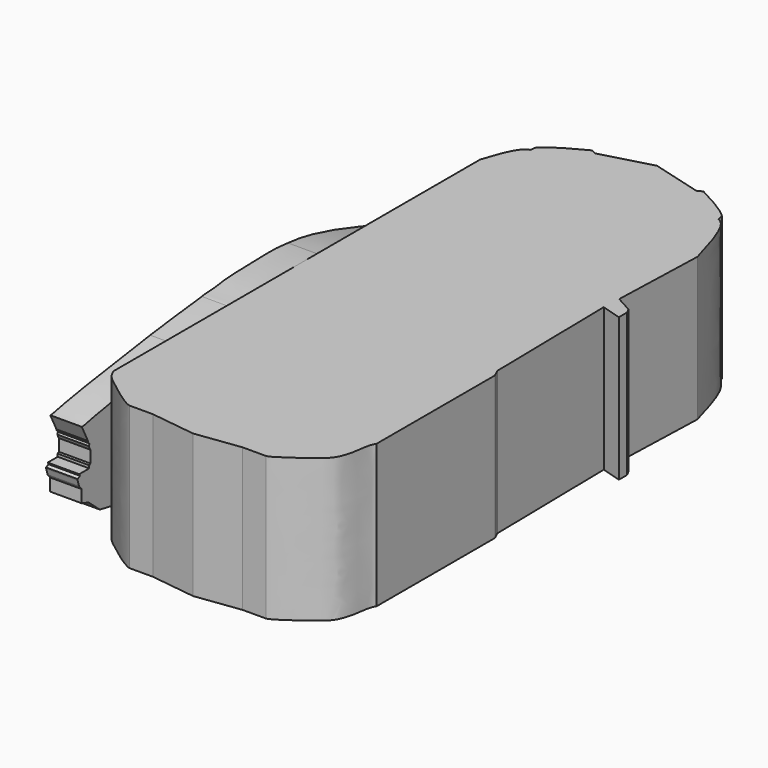
from build123d import *

# Parameters (mm, degrees)
F0_W     = 464.551
F0_H     = 113.6
F1_DEPTH = 113.25
F2_DEPTH = 113.25
F4_DEPTH = 25
F6_DEPTH = 1000


with BuildPart() as f1:
    # F0 (on Right) → F1 (new body)
    with BuildSketch(Plane.YZ):
        with Locations((0, 56.8)):
            Rectangle(F0_W, F0_H)
    extrude(amount=F1_DEPTH)

    # F2 (add): a face of the model
    f2_faces = [f1.faces().sort_by_distance(p)[0] for p in [
        (0, 0, 56.8),
    ]]
    extrude(f2_faces, amount=F2_DEPTH)

    # F3 (on face) → F4 (cut)
    with BuildSketch(Plane(origin=(-113.25, 0, 0), x_dir=(0, -1, 0), z_dir=(-1, 0, 0))):
        with BuildLine():
            Line((-232.2755, 113.6), (-232.2755, 32.8185763762))
            add(Edge.make_bspline(
                [(-232.2755, 32.8185763762), (-231.8790980509, 34.173098972), (-231.4615017526, 35.2897108989), (-231.1046542652, 36.061558603)],
                knots=[0.3164856699, 0.3164856699, 0.3164856699, 0.3164856699, 0.340416374, 0.340416374, 0.340416374, 0.340416374], degree=3))
            add(Edge.make_bspline(
                [(-231.1046542652, 36.061558603), (-231.1037416795, 36.0635324916), (-231.1028294911, 36.0655041254), (-231.1019176999, 36.0674735084)],
                knots=[0.340416374, 0.340416374, 0.340416374, 0.340416374, 0.3404775733, 0.3404775733, 0.3404775733, 0.3404775733], degree=3))
            add(Edge.make_bspline(
                [(-231.1019176999, 36.0674735084), (-230.6559874539, 37.3781955492), (-230.2235967105, 37.6932665807), (-229.7431129588, 38.2673442747), (-229.7240369276, 38.2904159632)],
                knots=[0.3710065635, 0.3710065635, 0.3710065635, 0.3710065635, 0.408928644, 0.410487131, 0.410487131, 0.410487131, 0.410487131], degree=3))
            add(Edge.make_bspline(
                [(-229.7240369276, 38.2904159632), (-229.3831871996, 38.9468266155), (-228.9939173404, 40.7418408458), (-222.7621322692, 45.1945330228), (-218.9446701646, 47.5596041628)],
                knots=[0.3837612534, 0.3837612534, 0.3837612534, 0.3837612534, 0.4345564552, 0.4775666683, 0.4775666683, 0.4775666683, 0.4775666683], degree=3))
            add(Edge.make_bspline(
                [(-218.9446701646, 47.5596041628), (-201.1108713778, 59.1756051595), (-159.2165627136, 79.5233669449), (-124.8394856244, 78.5623382324)],
                knots=[0.5003760226, 0.5003760226, 0.5003760226, 0.5003760226, 0.7066174583, 0.7066174583, 0.7066174583, 0.7066174583], degree=3))
            Line((-124.8394856244, 78.5623382324), (-124.8128838181, 78.5711071926))
            add(Edge.make_bspline(
                [(-124.8128838181, 78.5711071926), (-95.4129047028, 89.3393301028), (-52.7253294089, 104.695750439), (-18.6634613097, 111.2791553675), (-8.6977606118, 111.9964196387)],
                knots=[0, 0, 0, 0, 0.4399174375, 0.6645176817, 0.6645176817, 0.6645176817, 0.6645176817], degree=3))
            add(Edge.make_bspline(
                [(-8.6977606118, 111.9964196387), (2.6332697065, 113.6), (20.4424923427, 112.7872208771), (35.963276732, 112.6549982749), (45.5451939753, 112.3018279721), (56.6888041617, 111.6409761871), (64.2975464247, 109.951929701), (75.0365459893, 109.9324073647), (76.5711785486, 109.2785894871)],
                knots=[0, 0, 0, 0, 0.2490636409, 0.4235691057, 0.5634534133, 0.7107894117, 0.8474028434, 1, 1, 1, 1], degree=3))
            add(Edge.make_bspline(
                [(76.5711785486, 109.2785894871), (98.8196080664, 107.0355331865), (101.2230982613, 106.3033664287), (121.0916796929, 104.1045469497), (127.9400074251, 103.1173849293)],
                knots=[0, 0, 0, 0, 0.350874071, 0.5612199162, 0.5612199162, 0.5612199162, 0.5612199162], degree=3))
            add(Edge.make_bspline(
                [(127.9400074251, 103.1173849293), (153.8156108236, 99.4933517824), (189.8635745439, 94.1924701653), (199.3642186335, 92.2866301463), (217.3858562933, 89.420523582), (224.3752265839, 87.4593358123), (226.7716812547, 87.4656452566), (227.0337724394, 87.4753445387)],
                knots=[0, 0, 0, 0, 0.3930552732, 0.5481620816, 0.755041436, 0.9024722065, 0.9211456239, 0.9211456239, 0.9211456239, 0.9211456239], degree=3))
            Line((227.0337724394, 87.4753445387), (220.8725305078, 75.1084685326))
            Line((220.8725305078, 75.1084685326), (220.8725305078, 74.2925181985))
            Line((220.8725305078, 74.2925181985), (219.4038273609, 72.7422088385))
            Line((219.4038273609, 72.7422088385), (220.1381863869, 71.1918994784))
            Line((220.1381863869, 71.1918994784), (218.5948135174, 68.0700615048))
            Line((218.5948135174, 68.0700615048), (218.5948135174, 58.5093386471))
            Line((218.5948135174, 58.5093386471), (219.6228446281, 57.5841069222))
            Line((219.6228446281, 57.5841069222), (219.6228446281, 55.4252304137))
            Line((219.6228446281, 55.4252304137), (225.688257984, 55.4252304137))
            Line((225.688257984, 55.4252304137), (229.594791106, 55.4252304137))
            Line((229.594791106, 55.4252304137), (228.8092614925, 53.9363473654))
            Line((228.8092614925, 53.9363473654), (231.2004830437, 52.6747470382))
            Line((231.2004830437, 52.6747470382), (231.2004830437, 51.8779531121))
            Line((231.2004830437, 51.8779531121), (229.7012301004, 47.0750369132))
            Line((229.7012301004, 47.0750369132), (227.1657975233, 44.0031215549))
            Line((227.1657975233, 44.0031215549), (227.1657975233, 34.1228358448))
            Line((227.1657975233, 34.1228358448), (220.304498247, 31.9272167981))
            Line((220.304498247, 31.9272167981), (209.0519459761, 22.3213806748))
            Line((209.0519459761, 22.3213806748), (184.955375434, 17.8825389594))
            Line((184.955375434, 17.8825389594), (181.8208045852, 17.8825389594))
            add(Edge.make_bspline(
                [(109.7462345314, 11.3512530682), (105.13303124, 21.9971068237), (102.3295920912, 31.0067949184), (104.3007691763, 39.3500479436), (106.5787886857, 48.4665274974), (109.1198933454, 54.6206926313), (110.6540323122, 58.1162692133), (114.1247970317, 64.2584038543), (121.206458876, 69.1007924931), (128.0023361028, 72.5621948893), (135.7815625135, 75.1533703094), (158.4659606039, 76.2432867824), (173.9848172528, 69.3513817398), (182.8990728751, 48.3394334811), (186.6540110233, 40.7480202803), (182.5457507186, 21.0076564597), (181.8208045852, 17.8825389594)],
                knots=[0, 0, 0, 0, 0.0987938644, 0.1562912272, 0.2214221262, 0.2754761052, 0.3164249447, 0.3714453076, 0.4337725763, 0.4910116539, 0.5514503521, 0.6509165337, 0.7371979116, 0.8298327622, 0.929885825, 0.9556923225, 0.9556923225, 0.9556923225, 0.9556923225], degree=3))
            Line((109.7462345314, 11.3512530682), (-44.88848494, 8.9413357289))
            add(Edge.make_bspline(
                [(-44.88848494, 8.9413357289), (-43.1857559899, 5.9007342453), (-41.5231174, 2.9081292823), (-39.890128567, 0)],
                knots=[0.9375411424, 0.9375411424, 0.9375411424, 0.9375411424, 0.959328761, 0.959328761, 0.959328761, 0.959328761], degree=3))
            Line((-39.890128567, 0), (182.4303716421, 0))
            Line((182.4303716421, 0), (232.2755, 0))
            Line((232.2755, 0), (232.2755, 113.6))
            Line((232.2755, 113.6), (-232.2755, 113.6))
        make_face()
        with BuildLine():
            add(Edge.make_bspline(
                [(-164.6185908859, 5.2917431583), (-165.0713665181, 6.1458001934), (-165.5417803562, 7.0626109679), (-165.9595008133, 7.8887262308)],
                knots=[0.0253739484, 0.0253739484, 0.0253739484, 0.0253739484, 0.0325818946, 0.0325818946, 0.0325818946, 0.0325818946], degree=3))
            add(Edge.make_bspline(
                [(-164.6185908829, 5.2917431614), (-176.0597302488, 5.0024554897), (-221.4994853953, -2.2050957763), (-231.4882447651, 12.8488706649), (-232.2755, 14.7370494299)],
                knots=[0.0067884722, 0.0067884722, 0.0067884722, 0.0067884722, 0.2079627726, 0.2341336285, 0.2341336285, 0.2341336285, 0.2341336285], degree=3))
            Line((-232.2755, 14.7370494299), (-232.2755, 0))
            Line((-232.2755, 0), (-199.7243613005, 0))
            Line((-199.7243613005, 0), (-108.776524663, 0))
            add(Edge.make_bspline(
                [(-99.5009951625, 8.0902226298), (-100.0590209927, 7.5668730715), (-101.5069269475, 6.5632143557), (-103.3306144836, 6.7731347239), (-108.7701587892, 1.0011318839), (-108.776524663, 0)],
                knots=[0.9080949913, 0.9080949913, 0.9080949913, 0.9080949913, 0.9266826271, 0.9527213106, 1, 1, 1, 1], degree=3))
            add(Edge.make_bspline(
                [(-165.999836251, 7.9685384826), (-166.1315589651, 8.2293162171), (-168.3484257522, 12.6415430944), (-167.9805882713, 12.4600804675), (-169.7120256252, 17.9777869169), (-169.9426153794, 22.5907371267), (-169.5424098093, 28.9978956361), (-168.7921487837, 37.5297393179), (-166.0332983923, 49.9674844075), (-151.3616999612, 63.434506998), (-134.8432776987, 68.1280958415), (-117.8900740705, 65.973738886), (-105.2585534529, 57.8915639024), (-99.8095863375, 46.4784476464), (-97.2456192191, 38.6154807096), (-96.7354298507, 35.5495889525), (-95.4008258624, 29.1857470823), (-94.3373664851, 24.3061446971), (-95.2367782113, 18.2710500862), (-97.0664400304, 13.2465953537), (-97.7713663779, 9.980297143), (-99.1001790926, 8.4661315964), (-99.5009951625, 8.0902226298)],
                knots=[0.0328148598, 0.0328148598, 0.0328148598, 0.0328148598, 0.0351068846, 0.0730884918, 0.1078890541, 0.1446769101, 0.1863042014, 0.2349017732, 0.2935240518, 0.3663928625, 0.4352730595, 0.5031486338, 0.5664856863, 0.6257751938, 0.6724005796, 0.7019430205, 0.7436099057, 0.781676286, 0.8223597691, 0.8611079585, 0.894743955, 0.9080949913, 0.9080949913, 0.9080949913, 0.9080949913], degree=3))
            add(Edge.make_bspline(
                [(-165.9595008133, 7.8887262308), (-165.9730017954, 7.9154267842), (-165.9864477329, 7.9420325951), (-165.999836251, 7.9685384826)],
                knots=[0.0325818946, 0.0325818946, 0.0325818946, 0.0325818946, 0.0328148598, 0.0328148598, 0.0328148598, 0.0328148598], degree=3))
        make_face()
        with BuildLine():
            add(Edge.make_bspline(
                [(-163.5608168843, 5.2993261556), (-163.8792031032, 5.3043338554), (-164.2325184235, 5.3015049516), (-164.6185908829, 5.2917431614)],
                knots=[0, 0, 0, 0, 0.0067884722, 0.0067884722, 0.0067884722, 0.0067884722], degree=3))
            add(Edge.make_bspline(
                [(-163.5608168843, 5.2993261556), (-161.649380445, 0.0563780767), (-163.0246964147, 2.285228034), (-164.6185908859, 5.2917431583)],
                knots=[0, 0, 0, 0, 0.0253739484, 0.0253739484, 0.0253739484, 0.0253739484], degree=3))
        make_face(mode=Mode.SUBTRACT)
        with BuildLine():
            Line((-47.060206555, 8.9074903571), (-99.5009951625, 8.0902226298))
            add(Edge.make_bspline(
                [(-99.5009951625, 8.0902226298), (-100.0590209927, 7.5668730715), (-101.5069269475, 6.5632143557), (-103.3306144836, 6.7731347239), (-108.7701587892, 1.0011318839), (-108.776524663, 0)],
                knots=[0.9080949913, 0.9080949913, 0.9080949913, 0.9080949913, 0.9266826271, 0.9527213106, 1, 1, 1, 1], degree=3))
            Line((-108.776524663, 0), (-42.181071883, 0))
            add(Edge.make_bspline(
                [(-47.060206555, 8.9074903571), (-45.4160903787, 5.8952523745), (-43.7940471019, 2.9154941638), (-42.181071883, 0)],
                knots=[0.9352203433, 0.9352203433, 0.9352203433, 0.9352203433, 0.9579142214, 0.9579142214, 0.9579142214, 0.9579142214], degree=3))
        make_face()
        with BuildLine():
            add(Edge.make_bspline(
                [(-164.6185908829, 5.2917431614), (-176.0597302488, 5.0024554897), (-221.4994853953, -2.2050957763), (-231.4882447651, 12.8488706649), (-232.2755, 14.7370494299)],
                knots=[0.0067884722, 0.0067884722, 0.0067884722, 0.0067884722, 0.2079627726, 0.2341336285, 0.2341336285, 0.2341336285, 0.2341336285], degree=3))
            add(Edge.make_bspline(
                [(-164.6185908859, 5.2917431583), (-165.0713665181, 6.1458001934), (-165.5417803562, 7.0626109679), (-165.9595008133, 7.8887262308)],
                knots=[0.0253739484, 0.0253739484, 0.0253739484, 0.0253739484, 0.0325818946, 0.0325818946, 0.0325818946, 0.0325818946], degree=3))
            Line((-165.9595008133, 7.8887262308), (-173.761184881, 7.8887262308))
            add(Edge.make_bspline(
                [(-173.761184881, 7.8887262308), (-184.52015401, 6.7813550005), (-212.0861099631, 1.0960000393), (-224.4535929193, 8.6120162565)],
                knots=[0.0748722313, 0.0748722313, 0.0748722313, 0.0748722313, 0.2385609184, 0.2385609184, 0.2385609184, 0.2385609184], degree=3))
            add(Edge.make_bspline(
                [(-224.4535929198, 8.6120162548), (-225.593511103, 8.6582821597), (-226.9193272524, 8.9787715082), (-228.5662179841, 10.1463577013), (-228.0852725306, 10.5369179466), (-227.5320876257, 11.1132782623)],
                knots=[0.0190189348, 0.0190189348, 0.0190189348, 0.0190189348, 0.1288080398, 0.2164411512, 0.2955399174, 0.2955399174, 0.2955399174, 0.2955399174], degree=3))
            add(Edge.make_bspline(
                [(-227.5320876257, 11.1132782623), (-229.4142893106, 13.1628592742), (-230.626158224, 15.7357057729), (-231.3651247853, 18.4617653178)],
                knots=[0.2540536411, 0.2540536411, 0.2540536411, 0.2540536411, 0.287279567, 0.287279567, 0.287279567, 0.287279567], degree=3))
            add(Edge.make_bspline(
                [(-231.3651247856, 18.4617653194), (-231.6664931574, 18.3945211663), (-231.970246093, 18.3269098965), (-232.2755, 18.2591101898)],
                knots=[0.904683008, 0.904683008, 0.904683008, 0.904683008, 0.9170355344, 0.9170355344, 0.9170355344, 0.9170355344], degree=3))
            Line((-232.2755, 18.2591101898), (-232.2755, 14.7370494299))
        make_face()
        with BuildLine():
            add(Edge.make_bspline(
                [(-231.3651247853, 18.4617653178), (-231.8634715688, 20.3001746276), (-232.1467456858, 22.2082641541), (-232.2755, 24.0725370259)],
                knots=[0.287279567, 0.287279567, 0.287279567, 0.287279567, 0.30968658, 0.30968658, 0.30968658, 0.30968658], degree=3))
            add(Edge.make_bspline(
                [(-219.9768019121, 22.3368026759), (-220.4194158688, 22.4551950684), (-222.5269750091, 20.7593592711), (-222.0798182071, 20.5782839942), (-226.6219868008, 19.5200989952), (-231.3651247856, 18.4617653194)],
                knots=[0.5724422355, 0.5724422355, 0.5724422355, 0.5724422355, 0.6920254287, 0.7102706449, 0.904683008, 0.904683008, 0.904683008, 0.904683008], degree=3))
            add(Edge.make_bspline(
                [(-231.1042252985, 36.0606825889), (-230.5188300394, 34.8653239168), (-228.1407765352, 30.8516739145), (-225.1993287881, 26.8897443239), (-222.8176913923, 24.1323083158), (-220.2737508162, 22.4397358959), (-219.9768019121, 22.3368026759)],
                knots=[5.26887e-05, 5.26887e-05, 5.26887e-05, 5.26887e-05, 0.2157019808, 0.4186074107, 0.6166635747, 0.7051916224, 0.7051916224, 0.7051916224, 0.7051916224], degree=3))
            add(Edge.make_bspline(
                [(-232.2755, 29.1774376338), (-232.079015574, 32.1619360955), (-231.574978086, 34.6715181224), (-231.1052089772, 36.0577842723), (-231.1042252985, 36.0606825889)],
                knots=[0.3310073569, 0.3310073569, 0.3310073569, 0.3310073569, 0.3708575256, 0.3709411582, 0.3709411582, 0.3709411582, 0.3709411582], degree=3))
            Line((-232.2755, 29.1774376338), (-232.2755, 24.0725370259))
        make_face()
        with BuildLine():
            add(Edge.make_bspline(
                [(-173.761184881, 7.8887262308), (-184.52015401, 6.7813550005), (-212.0861099631, 1.0960000393), (-224.4535929193, 8.6120162565)],
                knots=[0.0748722313, 0.0748722313, 0.0748722313, 0.0748722313, 0.2385609184, 0.2385609184, 0.2385609184, 0.2385609184], degree=3))
            Line((-173.761184881, 7.8887262308), (-214.1551375389, 7.8887262308))
            Line((-214.1551375389, 7.8887262308), (-223.8230854273, 8.5997134447))
            add(Edge.make_bspline(
                [(-223.8230854273, 8.5997134447), (-224.0465712552, 8.5999469107), (-224.2561231466, 8.6040015412), (-224.4535929198, 8.6120162548)],
                knots=[0, 0, 0, 0, 0.0190189348, 0.0190189348, 0.0190189348, 0.0190189348], degree=3))
        make_face()
        with BuildLine():
            add(Edge.make_bspline(
                [(-218.9446701646, 47.5596041628), (-200.5086110348, 58.9814834606), (-159.678620058, 77.9481915129), (-126.6516175068, 77.9649911165)],
                knots=[0.4775666683, 0.4775666683, 0.4775666683, 0.4775666683, 0.6852802774, 0.6852802774, 0.6852802774, 0.6852802774], degree=3))
            Line((-126.6516175068, 77.9649911165), (-124.8394856244, 78.5623382324))
            add(Edge.make_bspline(
                [(-218.9446701646, 47.5596041628), (-201.1108713778, 59.1756051595), (-159.2165627136, 79.5233669449), (-124.8394856244, 78.5623382324)],
                knots=[0.5003760226, 0.5003760226, 0.5003760226, 0.5003760226, 0.7066174583, 0.7066174583, 0.7066174583, 0.7066174583], degree=3))
        make_face()
        with BuildLine():
            add(Edge.make_bspline(
                [(-219.9768019121, 22.3368026759), (-220.4194158688, 22.4551950684), (-222.5269750091, 20.7593592711), (-222.0798182071, 20.5782839942), (-226.6219868008, 19.5200989952), (-231.3651247856, 18.4617653194)],
                knots=[0.5724422355, 0.5724422355, 0.5724422355, 0.5724422355, 0.6920254287, 0.7102706449, 0.904683008, 0.904683008, 0.904683008, 0.904683008], degree=3))
            add(Edge.make_bspline(
                [(-227.5320876257, 11.1132782623), (-229.4142893106, 13.1628592742), (-230.626158224, 15.7357057729), (-231.3651247853, 18.4617653178)],
                knots=[0.2540536411, 0.2540536411, 0.2540536411, 0.2540536411, 0.287279567, 0.287279567, 0.287279567, 0.287279567], degree=3))
            add(Edge.make_bspline(
                [(-227.5320876257, 11.1132782623), (-227.400035455, 11.250862694), (-225.2045570672, 13.5818888158), (-219.0909408032, 21.9856806014), (-219.9598966124, 22.3312334306)],
                knots=[0.2955399174, 0.2955399174, 0.2955399174, 0.2955399174, 0.3144217844, 0.5708529783, 0.5708529783, 0.5708529783, 0.5708529783], degree=3))
            add(Edge.make_bspline(
                [(-219.9768019121, 22.3368026759), (-219.9709772016, 22.3347836208), (-219.9653405958, 22.3329261306), (-219.9598966124, 22.3312334306)],
                knots=[0.7051916224, 0.7051916224, 0.7051916224, 0.7051916224, 0.7069281172, 0.7069281172, 0.7069281172, 0.7069281172], degree=3))
        make_face()
        with BuildLine():
            Line((-44.88848494, 8.9413357289), (-47.060206555, 8.9074903571))
            add(Edge.make_bspline(
                [(-47.060206555, 8.9074903571), (-45.4160903787, 5.8952523745), (-43.7940471019, 2.9154941638), (-42.181071883, 0)],
                knots=[0.9352203433, 0.9352203433, 0.9352203433, 0.9352203433, 0.9579142214, 0.9579142214, 0.9579142214, 0.9579142214], degree=3))
            Line((-42.181071883, 0), (-39.890128567, 0))
            add(Edge.make_bspline(
                [(-44.88848494, 8.9413357289), (-43.1857559899, 5.9007342453), (-41.5231174, 2.9081292823), (-39.890128567, 0)],
                knots=[0.9375411424, 0.9375411424, 0.9375411424, 0.9375411424, 0.959328761, 0.959328761, 0.959328761, 0.959328761], degree=3))
        make_face()
        with BuildLine():
            add(Edge.make_bspline(
                [(-229.7240369276, 38.2904159632), (-229.3831871996, 38.9468266155), (-228.9939173404, 40.7418408458), (-222.7621322692, 45.1945330228), (-218.9446701646, 47.5596041628)],
                knots=[0.3837612534, 0.3837612534, 0.3837612534, 0.3837612534, 0.4345564552, 0.4775666683, 0.4775666683, 0.4775666683, 0.4775666683], degree=3))
            add(Edge.make_bspline(
                [(-229.7240369276, 38.2904159632), (-228.9042852099, 39.2818725235), (-227.5337806085, 41.62901739), (-220.9262489428, 46.2689076972), (-218.9446701646, 47.5596041628)],
                knots=[0.410487131, 0.410487131, 0.410487131, 0.410487131, 0.4774597805, 0.5003760226, 0.5003760226, 0.5003760226, 0.5003760226], degree=3))
        make_face()
        with BuildLine():
            add(Edge.make_bspline(
                [(-163.5608168843, 5.2993261556), (-161.649380445, 0.0563780767), (-163.0246964147, 2.285228034), (-164.6185908859, 5.2917431583)],
                knots=[0, 0, 0, 0, 0.0253739484, 0.0253739484, 0.0253739484, 0.0253739484], degree=3))
            add(Edge.make_bspline(
                [(-163.5608168843, 5.2993261556), (-163.8792031032, 5.3043338554), (-164.2325184235, 5.3015049516), (-164.6185908829, 5.2917431614)],
                knots=[0, 0, 0, 0, 0.0067884722, 0.0067884722, 0.0067884722, 0.0067884722], degree=3))
        make_face()
        with BuildLine():
            Line((-232.2755, 24.0725370259), (-232.2755, 18.2591101898))
            add(Edge.make_bspline(
                [(-231.3651247856, 18.4617653194), (-231.6664931574, 18.3945211663), (-231.970246093, 18.3269098965), (-232.2755, 18.2591101898)],
                knots=[0.904683008, 0.904683008, 0.904683008, 0.904683008, 0.9170355344, 0.9170355344, 0.9170355344, 0.9170355344], degree=3))
            add(Edge.make_bspline(
                [(-231.3651247853, 18.4617653178), (-231.8634715688, 20.3001746276), (-232.1467456858, 22.2082641541), (-232.2755, 24.0725370259)],
                knots=[0.287279567, 0.287279567, 0.287279567, 0.287279567, 0.30968658, 0.30968658, 0.30968658, 0.30968658], degree=3))
        make_face()
        with BuildLine():
            add(Edge.make_bspline(
                [(-232.2755, 32.8185763762), (-231.8790980509, 34.173098972), (-231.4615017526, 35.2897108989), (-231.1046542652, 36.061558603)],
                knots=[0.3164856699, 0.3164856699, 0.3164856699, 0.3164856699, 0.340416374, 0.340416374, 0.340416374, 0.340416374], degree=3))
            Line((-232.2755, 32.8185763762), (-232.2755, 29.1774376338))
            add(Edge.make_bspline(
                [(-232.2755, 29.1774376338), (-232.079015574, 32.1619360955), (-231.574978086, 34.6715181224), (-231.1052089772, 36.0577842723), (-231.1042252985, 36.0606825889)],
                knots=[0.3310073569, 0.3310073569, 0.3310073569, 0.3310073569, 0.3708575256, 0.3709411582, 0.3709411582, 0.3709411582, 0.3709411582], degree=3))
            add(Edge.make_bspline(
                [(-231.1046542652, 36.061558603), (-231.1045113145, 36.0612666504), (-231.1043683256, 36.0609746457), (-231.1042252985, 36.0606825889)],
                knots=[0, 0, 0, 0, 5.26887e-05, 5.26887e-05, 5.26887e-05, 5.26887e-05], degree=3))
        make_face()
        with BuildLine():
            add(Edge.make_bspline(
                [(-231.1046542652, 36.061558603), (-231.1037416795, 36.0635324916), (-231.1028294911, 36.0655041254), (-231.1019176999, 36.0674735084)],
                knots=[0.340416374, 0.340416374, 0.340416374, 0.340416374, 0.3404775733, 0.3404775733, 0.3404775733, 0.3404775733], degree=3))
            add(Edge.make_bspline(
                [(-231.1046542652, 36.061558603), (-231.1045113145, 36.0612666504), (-231.1043683256, 36.0609746457), (-231.1042252985, 36.0606825889)],
                knots=[0, 0, 0, 0, 5.26887e-05, 5.26887e-05, 5.26887e-05, 5.26887e-05], degree=3))
            add(Edge.make_bspline(
                [(-231.1042252985, 36.0606825889), (-231.1034560076, 36.0629492317), (-231.1026868082, 36.0652128694), (-231.1019176999, 36.0674735084)],
                knots=[0.3709411582, 0.3709411582, 0.3709411582, 0.3709411582, 0.3710065635, 0.3710065635, 0.3710065635, 0.3710065635], degree=3))
        make_face()
    extrude(amount=-F4_DEPTH, mode=Mode.SUBTRACT)

    # F5 (on face) → F6 (cut)
    with BuildSketch(Plane.XY.offset(113.6)):
        with BuildLine():
            add(Edge.make_bspline(
                [(98.4679684043, 150.3394693136), (92.97439072, 169.757588614), (87.4808130356, 189.1757079143), (80.6744733231, 195.6006419142)],
                knots=[0, 0, 0, 0, 0.3368607946, 0.3368607946, 0.3368607946, 0.3368607946], degree=3))
            Line((98.4679684043, 150.3394693136), (96.0445478559, 75.8095905185))
            Line((96.0445478559, 75.8095905185), (109.0543940663, 68.6613246799))
            Line((109.0543940663, 68.6613246799), (111.0559105873, 64.801260829))
            Line((111.0559105873, 64.801260829), (111.0559105873, 56.6522367299))
            Line((111.0559105873, 56.6522367299), (95.3297168016, 61.3700933754))
            Line((95.3297168016, 61.3700933754), (97.2140729427, -46.5304255486))
            Line((97.2140729427, -46.5304255486), (99.9343246222, -52.4809621274))
            Line((99.9343246222, -52.4809621274), (99.9343246222, -76.1131048203))
            Line((99.9343246222, -76.1131048203), (99.9343246222, -169.918820262))
            add(Edge.make_bspline(
                [(99.9343246222, -169.918820262), (97.4321093028, -173.1361196506), (96.4461367368, -184.839463119), (94.8029562123, -191.1416171803), (91.5085392438, -202.0027756883), (79.6216278842, -210.368717206), (70.4898681676, -217.4342853568), (68.7864026452, -218.5316457264), (60.0496902937, -224.5997639162), (56.7584149539, -225.4335582256)],
                knots=[0, 0, 0, 0, 0.1738619062, 0.2946412592, 0.4390511095, 0.6151901713, 0.7621131747, 0.8345390813, 1, 1, 1, 1], degree=3))
            Line((56.7584149539, -225.4335582256), (38.066457957, -225.4335582256))
            Line((38.066457957, -225.4335582256), (2.5091920979, -230.1075380633))
            Line((2.5091920979, -230.1075380633), (2.5091920979, -232.2755))
            Line((2.5091920979, -232.2755), (113.25, -232.2755))
            Line((113.25, -232.2755), (113.25, 232.2755))
            Line((113.25, 232.2755), (2.5091920979, 232.2755))
            Line((2.5091920979, 232.2755), (2.5091920979, 230.1537692547))
            Line((2.5091920979, 230.1537692547), (42.5678007305, 219.1463857889))
            Line((42.5678007305, 219.1463857889), (46.6435663402, 221.1842685938))
            add(Edge.make_bspline(
                [(46.6435663402, 221.1842685938), (58.3317560671, 215.0074812391), (70.0268380708, 208.83488258), (76.3282924907, 202.346215547)],
                knots=[0, 0, 0, 0, 0.3895306388, 0.3895306388, 0.3895306388, 0.3895306388], degree=3))
            add(Edge.make_bspline(
                [(76.3282924907, 202.346215547), (78.4723242857, 200.1384857915), (79.9919576532, 197.8941660801), (80.6744733231, 195.6006419142)],
                knots=[0.3895306388, 0.3895306388, 0.3895306388, 0.3895306388, 0.5220660853, 0.5220660853, 0.5220660853, 0.5220660853], degree=3))
        make_face()
        with BuildLine():
            add(Edge.make_bspline(
                [(80.6744733231, 195.6006419142), (79.5219646186, 196.6885676824), (78.3318161241, 197.4039500989), (77.0976543427, 197.6837068796)],
                knots=[0.3368607946, 0.3368607946, 0.3368607946, 0.3368607946, 0.3939009974, 0.3939009974, 0.3939009974, 0.3939009974], degree=3))
            add(Edge.make_bspline(
                [(76.3282924907, 202.346215547), (78.4723242857, 200.1384857915), (79.9919576532, 197.8941660801), (80.6744733231, 195.6006419142)],
                knots=[0.3895306388, 0.3895306388, 0.3895306388, 0.3895306388, 0.5220660853, 0.5220660853, 0.5220660853, 0.5220660853], degree=3))
            Line((76.3282924907, 202.346215547), (77.0976543427, 197.6837068796))
        make_face()
        with BuildLine():
            Line((-37.5494165346, 219.1463857889), (2.5091920979, 230.1537692547))
            Line((2.5091920979, 230.1537692547), (2.5091920979, 232.2755))
            Line((2.5091920979, 232.2755), (-88.25, 232.2755))
            Line((-88.25, 232.2755), (-88.25, 168.1774314647))
            add(Edge.make_bspline(
                [(-88.25, 168.1774314647), (-84.3878149029, 180.6419670643), (-80.3316975316, 191.1870397908), (-75.6560891272, 195.6006419142)],
                knots=[0.1054546014, 0.1054546014, 0.1054546014, 0.1054546014, 0.3368607946, 0.3368607946, 0.3368607946, 0.3368607946], degree=3))
            add(Edge.make_bspline(
                [(-71.3099082948, 202.346215547), (-73.4539400898, 200.1384857915), (-74.9735734573, 197.8941660801), (-75.6560891272, 195.6006419142)],
                knots=[0.3895306388, 0.3895306388, 0.3895306388, 0.3895306388, 0.5220660853, 0.5220660853, 0.5220660853, 0.5220660853], degree=3))
            add(Edge.make_bspline(
                [(-41.6251821443, 221.1842685938), (-53.3133718712, 215.0074812391), (-65.0084538749, 208.83488258), (-71.3099082948, 202.346215547)],
                knots=[0, 0, 0, 0, 0.3895306388, 0.3895306388, 0.3895306388, 0.3895306388], degree=3))
            Line((-41.6251821443, 221.1842685938), (-37.5494165346, 219.1463857889))
        make_face()
        with BuildLine():
            Line((2.5091920979, -232.2755), (2.5091920979, -230.1075380633))
            Line((2.5091920979, -230.1075380633), (-33.0480737612, -225.4335582256))
            Line((-33.0480737612, -225.4335582256), (-51.7400307581, -225.4335582256))
            add(Edge.make_bspline(
                [(-88.25, -195.7128689001), (-87.588972805, -197.4044979686), (-84.7389102072, -203.235291981), (-74.6032436883, -210.368717206), (-65.4714839717, -217.4342853568), (-63.7680184493, -218.5316457264), (-55.0313060978, -224.5997639162), (-51.7400307581, -225.4335582256)],
                knots=[0.3635117804, 0.3635117804, 0.3635117804, 0.3635117804, 0.4390511095, 0.6151901713, 0.7621131747, 0.8345390813, 1, 1, 1, 1], degree=3))
            Line((-88.25, -195.7128689001), (-88.25, -232.2755))
            Line((-88.25, -232.2755), (2.5091920979, -232.2755))
        make_face()
        with BuildLine():
            Line((-72.0792701468, 197.6837068796), (-71.3099082948, 202.346215547))
            add(Edge.make_bspline(
                [(-71.3099082948, 202.346215547), (-73.4539400898, 200.1384857915), (-74.9735734573, 197.8941660801), (-75.6560891272, 195.6006419142)],
                knots=[0.3895306388, 0.3895306388, 0.3895306388, 0.3895306388, 0.5220660853, 0.5220660853, 0.5220660853, 0.5220660853], degree=3))
            add(Edge.make_bspline(
                [(-75.6560891272, 195.6006419142), (-74.5035804227, 196.6885676824), (-73.3134319282, 197.4039500989), (-72.0792701468, 197.6837068796)],
                knots=[0.3368607946, 0.3368607946, 0.3368607946, 0.3368607946, 0.3939009974, 0.3939009974, 0.3939009974, 0.3939009974], degree=3))
        make_face()
    extrude(amount=-F6_DEPTH, mode=Mode.SUBTRACT)


solid = f1.part
